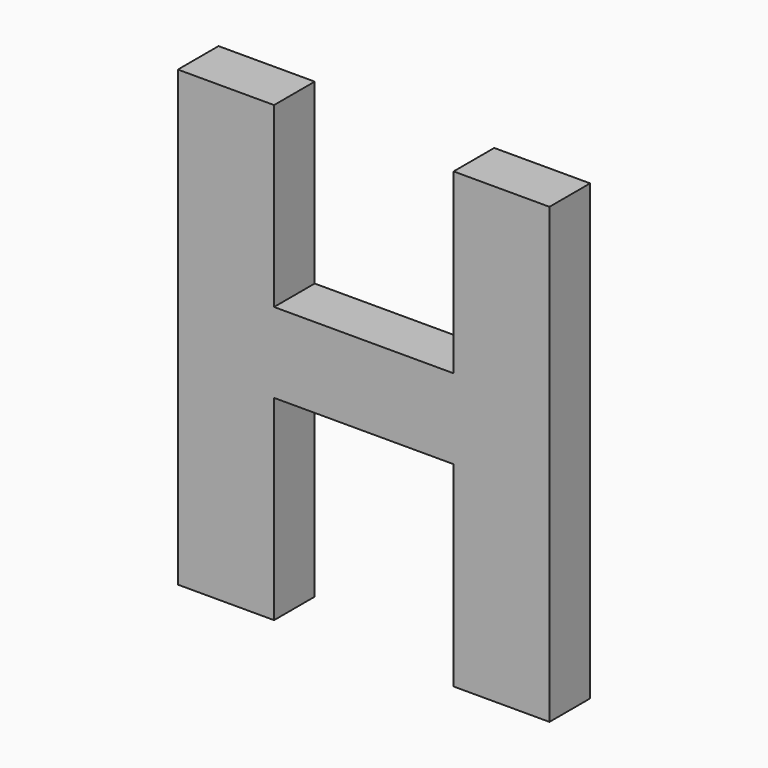
from build123d import *

# Parameters (mm, degrees)
F0_TEXT_SIZE = 62.5
F1_DEPTH     = 5


# Not quite as in the source:
# - Text() gives the source's letters only with a copy of the font that has no kerning and outlines rounded to 1/6400 em; it was checked with that copy


with BuildPart() as f1:
    # F0 (on Front) → F1 (new body)
    with BuildSketch(Plane.XZ):
        with Locations((-69.5111718623, 24.2597786663)):
            Text('H', F0_TEXT_SIZE, font='Open Sans', font_style=FontStyle.BOLD, text_align=(TextAlign.LEFT, TextAlign.BOTTOM))
    extrude(amount=F1_DEPTH)


solid = f1.part
